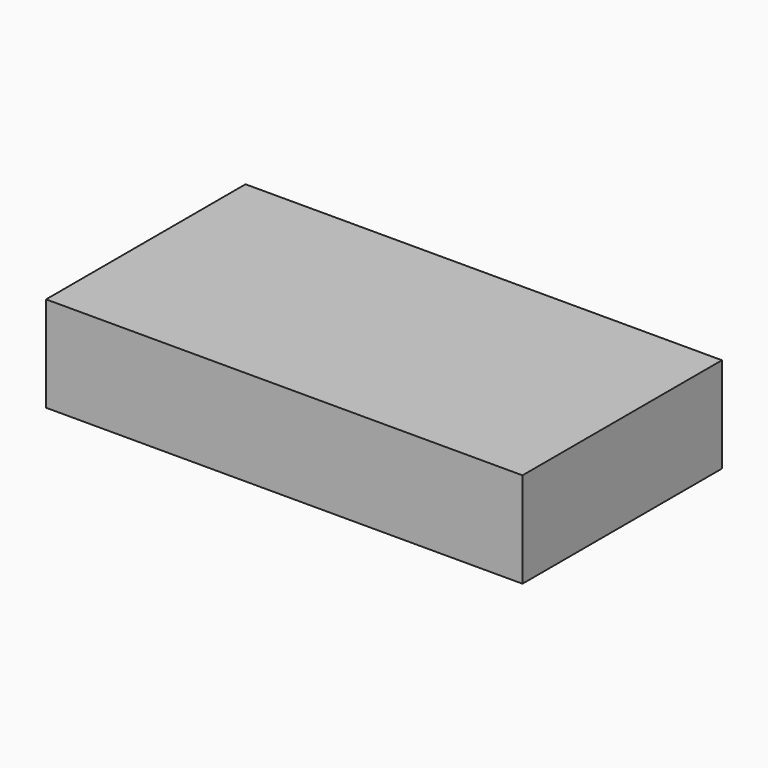
from build123d import *

# Parameters (mm, degrees)
F0_W     = 126.7785578966
F0_H     = 66.3399919868
F1_DEPTH = 25.4
F2_DEPTH = 159


# Not quite as in the source:
# - an extrude ends at something that could not be found from the text; its depth is read off the source's solid


with BuildPart() as f1:
    # F0 (on Top) → F1 (new body)
    with BuildSketch(Plane.XY):
        with Locations((1.9332244992, 33.1699959934)):
            Rectangle(F0_W, F0_H)
    extrude(amount=F1_DEPTH)

    # F2 (cut, through all): a face of the model
    f2_faces = [f1.faces().sort_by_distance(p)[0] for p in [
        (1.9332244992, 33.1699959934, 25.4),
    ]]
    extrude(f2_faces, amount=F2_DEPTH, mode=Mode.SUBTRACT)


solid = f1.part
